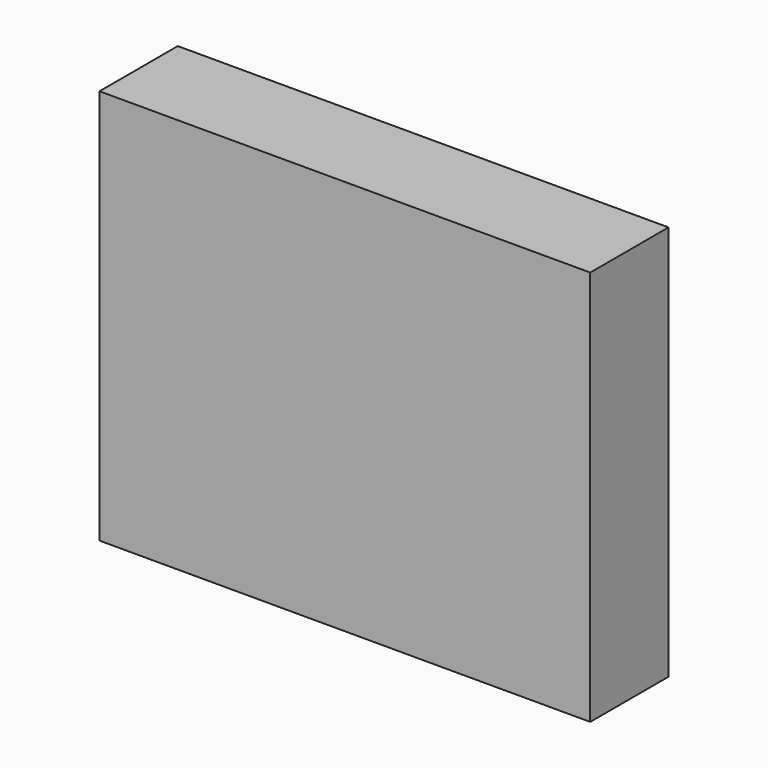
from build123d import *

# Parameters (mm, degrees)
F0_W     = 127.3891888559
F0_H     = 102.6856452227
F1_DEPTH = 25.4


# Not quite as in the source:
# - the program builds the solid bodies; features that only make, move or delete a surface that nothing else refers to are left out


with BuildPart() as f1:
    # F0 (on Front) → F1 (new body)
    with BuildSketch(Plane.XZ):
        with Locations((-6.7289490253, 3.9636306465)):
            Rectangle(F0_W, F0_H)
    extrude(amount=F1_DEPTH)


solid = f1.part
